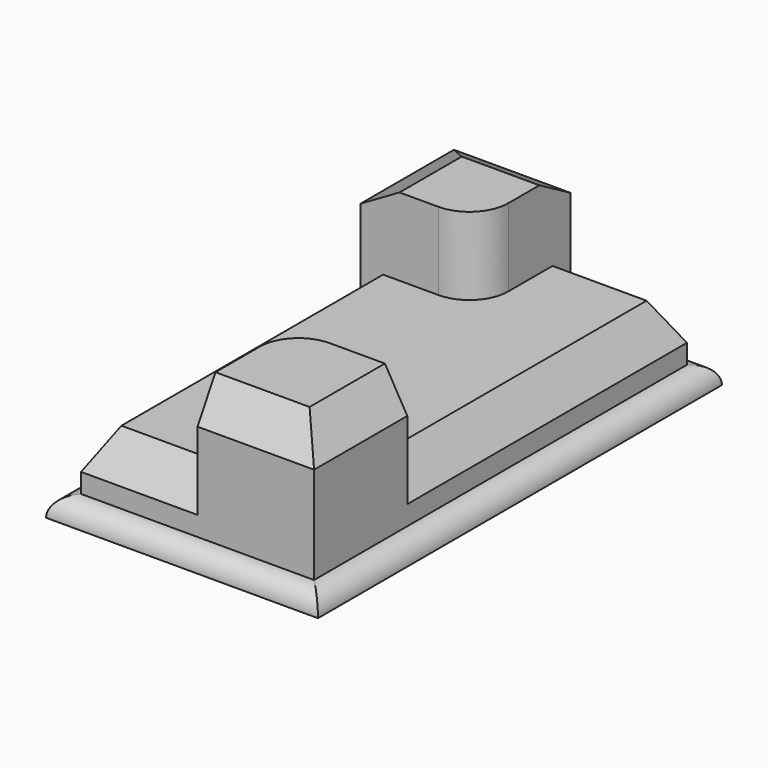
from build123d import *

# Parameters (mm, degrees)
F0_W        = 88.8999998465
F0_H        = 165.0999998465
F1_DEPTH    = 6.35
F2_DEPTH    = 25.4
F3_DEPTH    = 50.8
F4_R        = 6.34999
F5_C1_SIZE2 = 7.3323484187
F5_C1_SIZE  = 12.7
F5_C2_SIZE2 = 7.3323484187
F5_C2_SIZE  = 12.7
F5_C3_SIZE2 = 12.7
F5_C3_SIZE  = 7.3323484187
F5_C4_SIZE2 = 7.3323484187
F5_C4_SIZE  = 12.7
F5_C5_SIZE2 = 7.3323484187
F5_C5_SIZE  = 12.7
F5_C6_SIZE2 = 7.3323484187
F5_C6_SIZE  = 12.7
F6_SIZE2    = 7.3323484187
F6_SIZE     = 12.7
F6_2_SIZE2  = 7.3323484187
F6_2_SIZE   = 12.7


# Not quite as in the source:
# - a fillet or chamfer is up to 0.001 mm smaller than in the source, because OpenCascade refuses the exact size


with BuildPart() as f1:
    # F0 (on Top) → F1 (new body)
    with BuildSketch(Plane.XY):
        with Locations((38.1, -76.2)):
            Rectangle(F0_W, F0_H)
        Polygon((0, -38.1), (0, 0), (38.1, 0), (76.2, 0), (76.2, -114.3), (76.2, -152.4), (38.1, -152.4), (0, -152.4), align=None, mode=Mode.SUBTRACT)
    extrude(amount=F1_DEPTH)

    # F0 (on Top) → F2 (join)
    with BuildSketch(Plane.XY):
        with BuildLine():
            Line((76.2, 0), (38.1, 0))
            Line((38.1, 0), (38.1, -25.4))
            ThreePointArc((38.1, -25.4), (34.3802561211, -34.3802561211), (25.4, -38.1))
            Line((25.4, -38.1), (0, -38.1))
            Line((0, -38.1), (0, -152.4))
            Line((0, -152.4), (38.1, -152.4))
            Line((38.1, -152.4), (38.1, -127))
            ThreePointArc((38.1, -127), (41.8197438789, -118.0197438789), (50.8, -114.3))
            Line((50.8, -114.3), (76.2, -114.3))
            Line((76.2, -114.3), (76.2, 0))
        make_face()
    extrude(amount=F2_DEPTH)

    # F0 (on Top) → F3 (join)
    with BuildSketch(Plane.XY):
        with BuildLine():
            Line((38.1, 0), (0, 0))
            Line((0, 0), (0, -38.1))
            Line((0, -38.1), (25.4, -38.1))
            ThreePointArc((25.4, -38.1), (34.3802561211, -34.3802561211), (38.1, -25.4))
            Line((38.1, -25.4), (38.1, 0))
        make_face()
        with BuildLine():
            Line((76.2, -152.4), (76.2, -114.3))
            Line((76.2, -114.3), (50.8, -114.3))
            ThreePointArc((50.8, -114.3), (41.8197438789, -118.0197438789), (38.1, -127))
            Line((38.1, -127), (38.1, -152.4))
            Line((38.1, -152.4), (76.2, -152.4))
        make_face()
    extrude(amount=F3_DEPTH)

    # F4 (radius 6.35 in the source; OpenCascade refuses exactly that, so slightly less here)
    f4_edges = [f1.edges().sort_by_distance(p)[0] for p in [
        (38.1, -158.75, 6.35),
        (82.55, -76.2, 6.35),
        (-6.35, -76.2, 6.35),
        (38.1, 6.35, 6.35),
    ]]
    fillet(f4_edges, radius=F4_R)

    # F5: chamfer of 12.7 x 7.3323484187 on 6 edges, made by hand

    # F5_c1
    f5_c1_edges = [f1.edges().sort_by_distance(p)[0] for p in [
        (0, -95.25, 25.4),
    ]]
    f5_c1_side = f1.faces().sort_by_distance((0, -95.25, 25.2533530316))[0]
    chamfer(f5_c1_edges, length=F5_C1_SIZE, length2=F5_C1_SIZE2, reference=f5_c1_side)

    # F5_c2
    f5_c2_edges = [f1.edges().sort_by_distance(p)[0] for p in [
        (57.15, 0, 25.4),
    ]]
    f5_c2_side = f1.faces().sort_by_distance((57.15, 0, 25.2533530316))[0]
    chamfer(f5_c2_edges, length=F5_C2_SIZE, length2=F5_C2_SIZE2, reference=f5_c2_side)

    # F5_c3
    f5_c3_edges = [f1.edges().sort_by_distance(p)[0] for p in [
        (19.05, 0, 50.8),
    ]]
    f5_c3_side = f1.faces().sort_by_distance((19.05, 0, 50.6533530316))[0]
    chamfer(f5_c3_edges, length=F5_C3_SIZE, length2=F5_C3_SIZE2, reference=f5_c3_side)

    # F5_c4
    f5_c4_edges = [f1.edges().sort_by_distance(p)[0] for p in [
        (76.2, -60.8161742094, 25.4),
    ]]
    f5_c4_side = f1.faces().sort_by_distance((76.2, -60.8161742094, 25.2533530316))[0]
    chamfer(f5_c4_edges, length=F5_C4_SIZE, length2=F5_C4_SIZE2, reference=f5_c4_side)

    # F5_c5
    f5_c5_edges = [f1.edges().sort_by_distance(p)[0] for p in [
        (22.7161742094, -152.4, 25.4),
    ]]
    f5_c5_side = f1.faces().sort_by_distance((22.7161742094, -152.4, 25.2533530316))[0]
    chamfer(f5_c5_edges, length=F5_C5_SIZE, length2=F5_C5_SIZE2, reference=f5_c5_side)

    # F5_c6
    f5_c6_edges = [f1.edges().sort_by_distance(p)[0] for p in [
        (57.15, -152.4, 50.8),
    ]]
    f5_c6_side = f1.faces().sort_by_distance((57.15, -152.4, 50.6533530316))[0]
    chamfer(f5_c6_edges, length=F5_C6_SIZE, length2=F5_C6_SIZE2, reference=f5_c6_side)

    # F6
    f6_edges = [f1.edges().sort_by_distance(p)[0] for p in [
        (0, -25.4, 50.8),
    ]]
    f6_side = f1.faces().sort_by_distance((18.448591, -25.034136, 50.8))[0]
    chamfer(f6_edges, length=F6_SIZE, length2=F6_SIZE2, reference=f6_side)

    # F6#2
    f6_2_edges = [f1.edges().sort_by_distance(p)[0] for p in [
        (76.2, -129.683826, 50.8),
    ]]
    f6_2_side = f1.faces().sort_by_distance((76.2, -129.683826, 49.2125))[0]
    chamfer(f6_2_edges, length=F6_2_SIZE, length2=F6_2_SIZE2, reference=f6_2_side)


solid = f1.part
